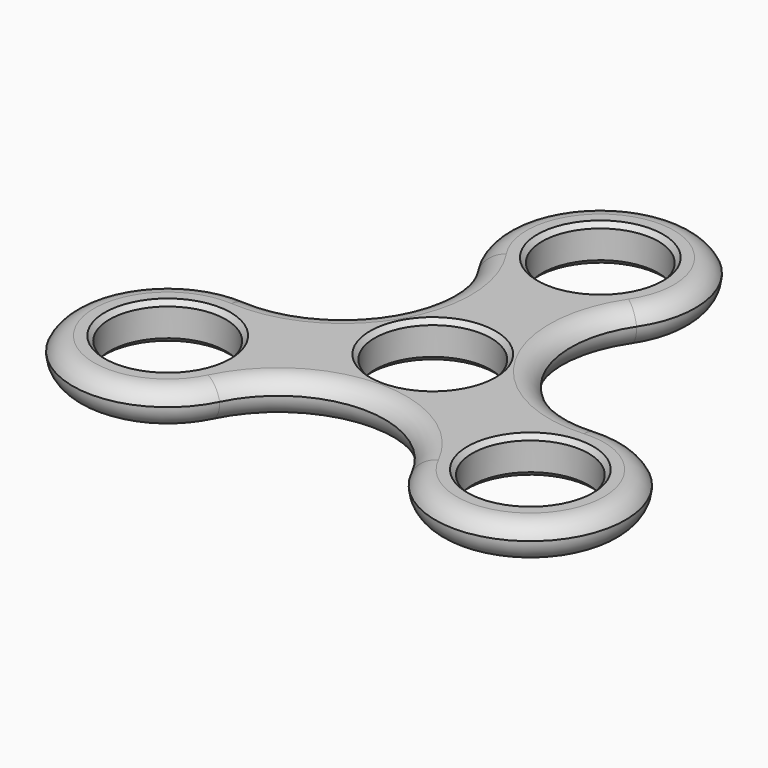
from build123d import *

# Parameters (mm, degrees)
F0_R         = 12.5
F1_DEPTH     = 4
F2_R         = 5.08
F3_T2_ANGLE  = 247.9325914863
F3_T4_ANGLE  = 127.9325914863
F3_T6_ANGLE  = 247.9325914863
F3_T8_ANGLE  = 127.9325914863
F3_T10_ANGLE = 247.9325914863
F3_T12_ANGLE = 127.9325914863
F4_SIZE      = 1
F5_SIZE      = 1


# Not quite as in the source:
# - a fillet or chamfer that OpenCascade refuses, or shapes differently, is made with other operations: its cross-section is extruded or revolved along the edge and cut away or added


with BuildPart() as f1:
    # F0 (on Top) → F1 (new body, symmetric)
    with BuildSketch(Plane.XY):
        with BuildLine():
            ThreePointArc((37.5585783682, -2.1271674207), (16.095780639, 9.2929032847), (16.9371081597, 33.5902667072))
            ThreePointArc((16.9371081597, 33.5902667072), (0, 65.421744456), (-16.9371081597, 33.5902667072))
            ThreePointArc((-16.9371081597, 33.5902667072), (-16.095780639, 9.2929032847), (-37.5585783682, -2.1271674207))
            ThreePointArc((-37.5585783682, -2.1271674207), (-56.6568926588, -32.710872228), (-20.6214702085, -31.4630992865))
            ThreePointArc((-20.6214702085, -31.4630992865), (0, -18.5858065695), (20.6214702085, -31.4630992865))
            ThreePointArc((20.6214702085, -31.4630992865), (56.6568926588, -32.710872228), (37.5585783682, -2.1271674207))
        make_face()
        with Locations((-38.9711431703, -22.5)):
            Circle(F0_R, mode=Mode.SUBTRACT)
        with Locations((38.9711431703, -22.5)):
            Circle(F0_R, mode=Mode.SUBTRACT)
        Circle(F0_R, mode=Mode.SUBTRACT)
        with Locations((0, 45)):
            Circle(F0_R, mode=Mode.SUBTRACT)
    extrude(amount=F1_DEPTH, both=True)

    # F2
    f2_edges = [f1.edges().sort_by_distance(p)[0] for p in [
        (-56.656893, -32.710872, -4),
        (0, -18.585807, -4),
    ]]
    fillet(f2_edges, radius=F2_R)

    # F3: fillet of radius 5.08 on 2 edges, made by hand

    # F3_s1 → F3_t2 (revolve, cut)
    with BuildSketch(Plane(origin=(-37.2320986027, 2.5815139741, 0), x_dir=(0, 0, 1), z_dir=(0.9976049119, -0.0691696444, 0))):
        with BuildLine():
            ThreePointArc((4, 9.3178987472), (3.2083096903, 6.5945184947), (1.08, 4.7199861774))
            Line((1.08, 4.7199861774), (4, 4.7199861774))
            Line((4, 4.7199861774), (4, 9.3178987472))
        make_face()
    revolve(axis=Axis((-38.9711431703, -22.5, 4), (0, 0, 1)), revolution_arc=F3_T2_ANGLE, mode=Mode.SUBTRACT)

    # F3_s3 → F3_t4 (revolve, cut)
    with BuildSketch(Plane(origin=(-20.8517059831, 30.9531862391, 0), x_dir=(0, 0, 1), z_dir=(-0.5587051252, 0.8293663745, 0))):
        with BuildLine():
            ThreePointArc((4, 9.3178987472), (3.2083096903, 6.5945184947), (1.08, 4.7199861774))
            Line((1.08, 4.7199861774), (4, 4.7199861774))
            Line((4, 4.7199861774), (4, 9.3178987472))
        make_face()
    revolve(axis=Axis((-35.9711297502, 20.7679414443, 4), (0, 0, -1)), revolution_arc=F3_T4_ANGLE, mode=Mode.SUBTRACT)

    # F3_s5 → F3_t6 (revolve, cut)
    with BuildSketch(Plane(origin=(20.8517059831, 30.9531862391, 0), x_dir=(0, 0, 1), z_dir=(-0.5587051252, -0.8293663745, 0))):
        with BuildLine():
            ThreePointArc((1.08, 4.7199861774), (3.2083096903, 6.5945184947), (4, 9.3178987472))
            Line((4, 9.3178987472), (4, 4.7199861774))
            Line((4, 4.7199861774), (1.08, 4.7199861774))
        make_face()
    revolve(axis=Axis((0, 45, 4), (0, 0, 1)), revolution_arc=F3_T6_ANGLE, mode=Mode.SUBTRACT)

    # F3_s7 → F3_t8 (revolve, cut)
    with BuildSketch(Plane(origin=(37.2320986027, 2.5815139741, 0), x_dir=(0, 0, 1), z_dir=(0.9976049119, 0.0691696444, 0))):
        with BuildLine():
            ThreePointArc((1.08, 4.7199861774), (3.2083096903, 6.5945184947), (4, 9.3178987472))
            Line((4, 9.3178987472), (4, 4.7199861774))
            Line((4, 4.7199861774), (1.08, 4.7199861774))
        make_face()
    revolve(axis=Axis((35.9711297502, 20.7679414443, 4), (0, 0, -1)), revolution_arc=F3_T8_ANGLE, mode=Mode.SUBTRACT)

    # F3_s9 → F3_t10 (revolve, cut)
    with BuildSketch(Plane(origin=(16.3803926196, -33.5347002132, 0), x_dir=(0, 0, 1), z_dir=(-0.4388997867, 0.8985360189, 0))):
        with BuildLine():
            ThreePointArc((4, 9.3178987472), (3.2083096903, 6.5945184947), (1.08, 4.7199861774))
            Line((1.08, 4.7199861774), (4, 4.7199861774))
            Line((4, 4.7199861774), (4, 9.3178987472))
        make_face()
    revolve(axis=Axis((38.9711431703, -22.5, 4), (0, 0, 1)), revolution_arc=F3_T10_ANGLE, mode=Mode.SUBTRACT)

    # F3_s11 → F3_t12 (revolve, cut)
    with BuildSketch(Plane(origin=(-16.3803926196, -33.5347002132, 0), x_dir=(0, 0, 1), z_dir=(-0.4388997867, -0.8985360189, 0))):
        with BuildLine():
            ThreePointArc((4, 9.3178987472), (3.2083096903, 6.5945184947), (1.08, 4.7199861774))
            Line((1.08, 4.7199861774), (4, 4.7199861774))
            Line((4, 4.7199861774), (4, 9.3178987472))
        make_face()
    revolve(axis=Axis((0, -41.5358828886, 4), (0, 0, -1)), revolution_arc=F3_T12_ANGLE, mode=Mode.SUBTRACT)

    # F4
    f4_edges = [f1.edges().sort_by_distance(p)[0] for p in [
        (-51.471143, -22.5, 4),
        (-12.5, 45, 4),
        (26.471143, -22.5, 4),
        (-12.5, 0, 4),
    ]]
    chamfer(f4_edges, length=F4_SIZE)

    # F5
    f5_edges = [f1.edges().sort_by_distance(p)[0] for p in [
        (-12.5, 0, -4),
        (-12.5, 45, -4),
        (-51.471143, -22.5, -4),
        (26.471143, -22.5, -4),
    ]]
    chamfer(f5_edges, length=F5_SIZE)


solid = f1.part
